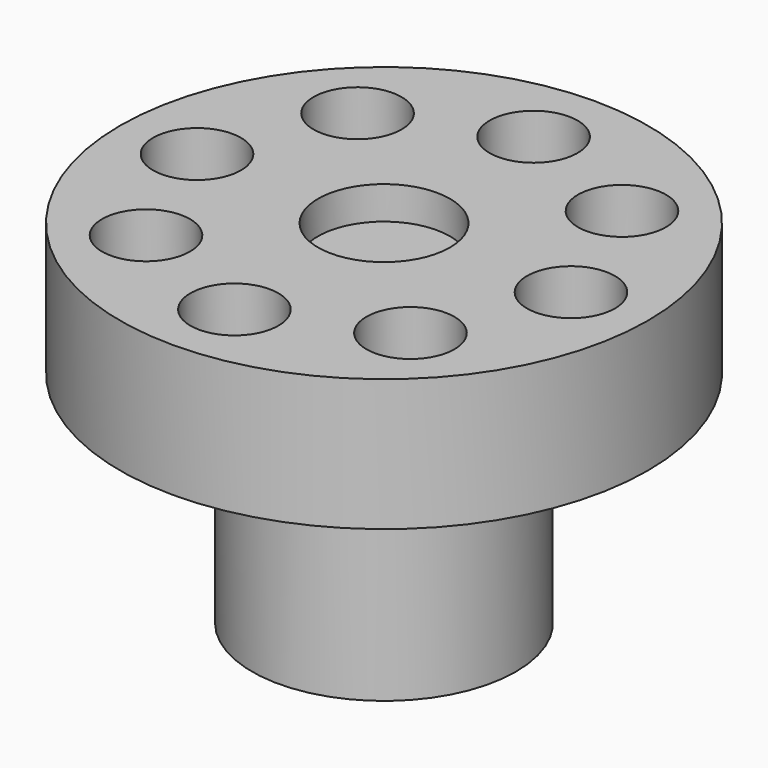
from build123d import *

# Parameters (mm, degrees)
F2_R            = 1
F3_DEPTH        = 3
F3_COPIES_COUNT = 8
F4_R            = 1.5
F5_DEPTH        = 0.75


# Not quite as in the source:
# - a pattern or mirror of a feature is missing from the dataset's text; its kind, count and spacing are read off the source's solid


with BuildPart() as f1:
    # F0 (on Front) → F1 (revolve)
    with BuildSketch(Plane.XZ):
        Polygon((0, 8), (0, 0), (3, 0), (3, 5), (6, 5), (6, 8), align=None)
    revolve(axis=Axis((0, 0, 4), (0, 0, -1)))

    # F2 (on face) → F3 (cut, through all)
    with BuildSketch(Plane.XY.offset(8)):
        with Locations((4.25, 0)):
            Circle(F2_R)
    f3 = extrude(amount=-F3_DEPTH, mode=Mode.SUBTRACT)

    # F3_copies: F3 ×8 about axis
    f3_copies_axis = Axis((0, 0, 0), (0, 0, 1))
    for i in range(1, F3_COPIES_COUNT):
        add(f3.rotate(f3_copies_axis, i * 360 / F3_COPIES_COUNT), mode=Mode.SUBTRACT)

    # F4 (on face) → F5 (cut)
    with BuildSketch(Plane.XY.offset(8)):
        Circle(F4_R)
    extrude(amount=-F5_DEPTH, mode=Mode.SUBTRACT)


solid = f1.part
